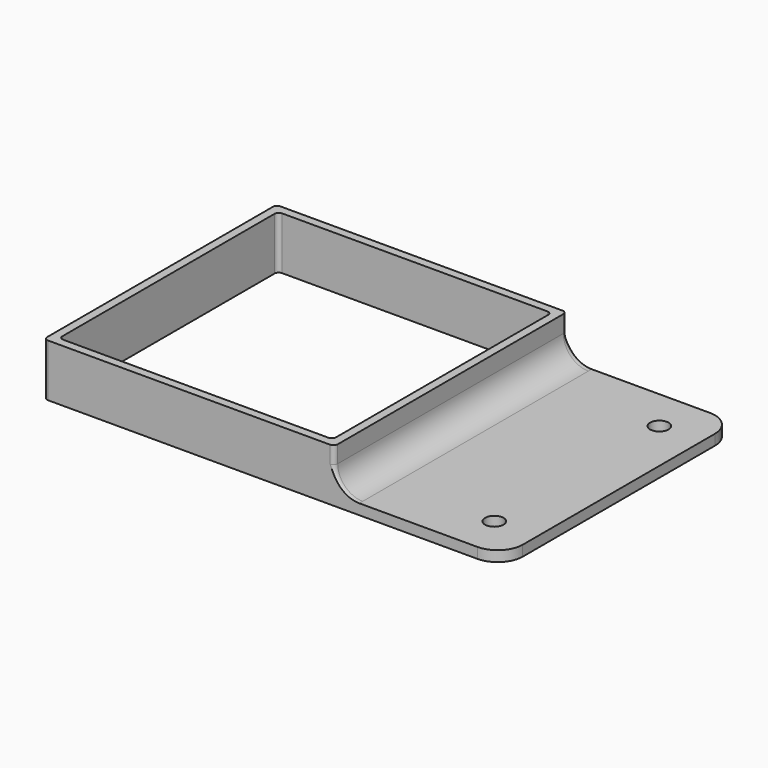
from build123d import *

# Parameters (mm, degrees)
F0_W         = 69
F0_H         = 69
F0_W_2       = 65
F0_H_2       = 65
F1_DEPTH     = 10
F0_W_3       = 40
F2_DEPTH     = 2.5
F3_R         = 1
F4_T1_DEPTH  = 67
F4_T6_ANGLE  = 359.64
F4_T12_ANGLE = 359.64
F4_T15_DEPTH = 32.5048284938
F5_D         = 4.4


# Not quite as in the source:
# - a fillet or chamfer that OpenCascade refuses, or shapes differently, is made with other operations: its cross-section is extruded or revolved along the edge and cut away or added


with BuildPart() as f1:
    # F0 (on Top) → F1 (new body)
    with BuildSketch(Plane.XY):
        Rectangle(F0_W, F0_H)
        Rectangle(F0_W_2, F0_H_2, mode=Mode.SUBTRACT)
    extrude(amount=F1_DEPTH)

    # F0 (on Top) → F2 (join)
    with BuildSketch(Plane.XY):
        with Locations((54.5, 0)):
            Rectangle(F0_W_3, F0_H)
        Rectangle(F0_W, F0_H)
        Rectangle(F0_W_2, F0_H_2, mode=Mode.SUBTRACT)
    extrude(amount=-F2_DEPTH)

    # F3
    f3_edges = [f1.edges().sort_by_distance(p)[0] for p in [
        (32.5, 32.5, 3.75),
        (-32.5, 32.5, 3.75),
        (-32.5, -32.5, 3.75),
        (32.5, -32.5, 3.75),
        (-34.5, 34.5, 3.75),
        (-34.5, -34.5, 3.75),
        (34.5, 34.5, 5),
        (34.5, -34.5, 5),
    ]]
    fillet(f3_edges, radius=F3_R)

    # F4: fillet of radius 6 on 3 edges, made by hand

    # F4_s2 → F4_t1 (join)
    with BuildSketch(Plane.XZ.offset(-33.5)):
        with BuildLine():
            ThreePointArc((40.5009656854, -0.0004), (36.2573593129, 1.7573593129), (34.4996, 6.0009656854))
            Line((34.4996, 6.0009656854), (33.8994634315, 6.0009656854))
            ThreePointArc((33.8994634315, 6.0009656854), (33.8998634315, 3.0004828427), (33.8998634315, 0))
            Line((33.8998634315, 0), (34.5, -0.6001365685))
            ThreePointArc((34.5, -0.6001365685), (37.5004828427, -0.6001365685), (40.5009656854, -0.6005365685))
            Line((40.5009656854, -0.6005365685), (40.5009656854, -0.0004))
        make_face()
    extrude(amount=F4_T1_DEPTH)


with BuildPart() as f4_tool4:
    # F4_s5 → F4_t6 (revolve)
    with BuildSketch(Plane(origin=(0.2118036776, -33.7091586585, 0), x_dir=(0, 0, 1), z_dir=(0.006283144, -0.9999802609, 0))):
        with BuildLine():
            ThreePointArc((6.0009656854, -34.2884534158), (1.7573593129, -36.0462127287), (-0.0004, -40.2898191013))
            Line((-0.0004, -40.2898191013), (-0.6005365685, -40.2898191013))
            ThreePointArc((-0.6005365685, -40.2898191013), (-0.6001365685, -37.2893362585), (-0.6001365685, -34.2888534158))
            Line((-0.6001365685, -34.2888534158), (0, -33.6887168473))
            ThreePointArc((0, -33.6887168473), (3.0004828427, -33.6887168473), (6.0009656854, -33.6883168473))
            Line((6.0009656854, -33.6883168473), (6.0009656854, -34.2884534158))
        make_face()
    revolve(axis=Axis((33.5, -33.5, 0), (0, 0, 1)), revolution_arc=F4_T6_ANGLE)

    split(bisect_by=Plane.XZ.offset(34.5), keep=Keep.BOTTOM)

    split(bisect_by=Plane.YZ.offset(32.5), keep=Keep.TOP)


with BuildPart() as f1_1:
    add(f1.part)

    # F4_t3: union F4_tool4
    add(f4_tool4.part)


with BuildPart() as f4_tool10:
    # F4_s11 → F4_t12 (revolve)
    with BuildSketch(Plane(origin=(0.2118036776, 33.7091586585, 0), x_dir=(0, 0, 1), z_dir=(0.006283144, 0.9999802609, 0))):
        with BuildLine():
            ThreePointArc((-0.0004, 40.2898191013), (1.7573593129, 36.0462127287), (6.0009656854, 34.2884534158))
            Line((6.0009656854, 34.2884534158), (6.0009656854, 33.6883168473))
            ThreePointArc((6.0009656854, 33.6883168473), (3.0004828427, 33.6887168473), (0, 33.6887168473))
            Line((0, 33.6887168473), (-0.6001365685, 34.2888534158))
            ThreePointArc((-0.6001365685, 34.2888534158), (-0.6001365685, 37.2893362585), (-0.6005365685, 40.2898191013))
            Line((-0.6005365685, 40.2898191013), (-0.0004, 40.2898191013))
        make_face()
    revolve(axis=Axis((33.5, 33.5, 0), (0, 0, -1)), revolution_arc=F4_T12_ANGLE)

    split(bisect_by=Plane.XZ.offset(-34.5), keep=Keep.TOP)

    split(bisect_by=Plane.YZ.offset(32.5), keep=Keep.TOP)


with BuildPart() as f1_2:
    add(f1_1.part)

    # F4_t9: union F4_tool10
    add(f4_tool10.part)

    # F4_s16 → F4_t15 (cut)
    with BuildSketch(Plane.XY.offset(-17.5024142469)):
        with BuildLine():
            ThreePointArc((68.4990343146, 34.5004), (72.7426406871, 32.7426406871), (74.5004, 28.4990343146))
            Line((74.5004, 28.4990343146), (75.1005365685, 28.4990343146))
            ThreePointArc((75.1005365685, 28.4990343146), (75.1001365685, 31.4995171573), (75.1001365685, 34.5))
            Line((75.1001365685, 34.5), (74.5, 35.1001365685))
            ThreePointArc((74.5, 35.1001365685), (71.4995171573, 35.1001365685), (68.4990343146, 35.1005365685))
            Line((68.4990343146, 35.1005365685), (68.4990343146, 34.5004))
        make_face()
        with BuildLine():
            ThreePointArc((68.4990343146, -34.5004), (72.7426406871, -32.7426406871), (74.5004, -28.4990343146))
            Line((74.5004, -28.4990343146), (75.1005365685, -28.4990343146))
            ThreePointArc((75.1005365685, -28.4990343146), (75.1001365685, -31.4995171573), (75.1001365685, -34.5))
            Line((75.1001365685, -34.5), (74.5, -35.1001365685))
            ThreePointArc((74.5, -35.1001365685), (71.4995171573, -35.1001365685), (68.4990343146, -35.1005365685))
            Line((68.4990343146, -35.1005365685), (68.4990343146, -34.5004))
        make_face()
    extrude(amount=F4_T15_DEPTH, mode=Mode.SUBTRACT)

    # F5 (through all)
    with Locations(Plane.XY):
        with Locations((64.5, -24.5), (64.5, 24.5)):
            Hole(F5_D / 2)


solid = f1_2.part
